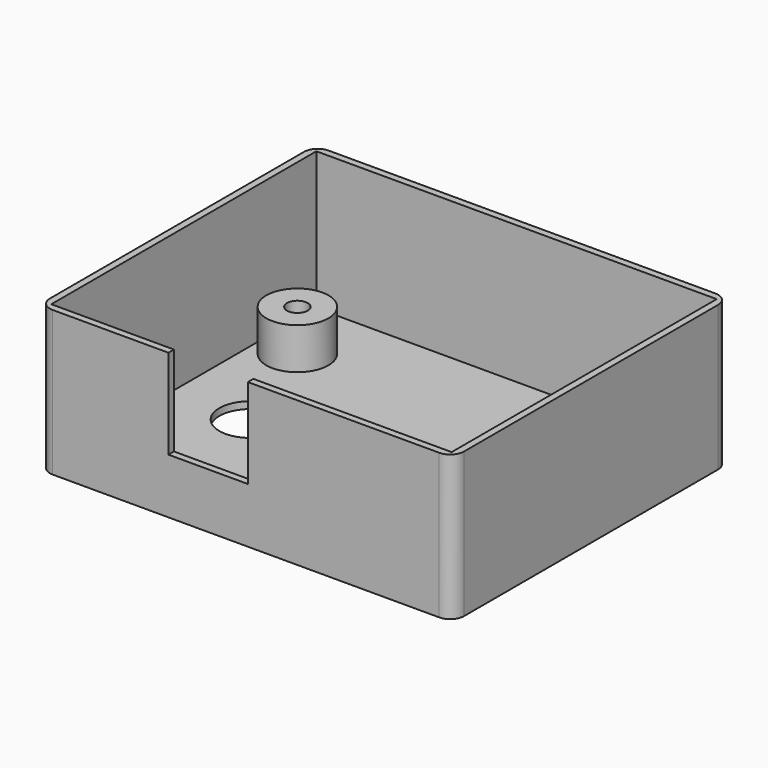
from build123d import *

# Parameters (mm, degrees)
F0_W      = 60
F0_H      = 50
F1_DEPTH  = 21
F2_W      = 58
F2_H      = 48
F3_DEPTH  = 20
F5_R      = 2
F6_R      = 4.5
F7_DEPTH  = 6
F10_W     = 11.5
F10_H     = 1
F11_DEPTH = 13
F12_W     = 2.5
F12_H     = 3.5
F13_DEPTH = 1
F14_R     = 4.5
F15_DEPTH = 1
F8_R      = 1.5
F16_DEPTH = 7
F9_R      = 1.5
F17_DEPTH = 7
F18_R     = 3.5
F18_R_2   = 1.5
F19_DEPTH = 1


with BuildPart() as f1:
    # F0 (on Top) → F1 (new body)
    with BuildSketch(Plane.XY):
        with Locations((-30, 25)):
            Rectangle(F0_W, F0_H)
    extrude(amount=F1_DEPTH)

    # F2 (on face) → F3 (cut)
    with BuildSketch(Plane.XY.offset(21)):
        with Locations((-30, 25)):
            Rectangle(F2_W, F2_H)
    extrude(amount=-F3_DEPTH, mode=Mode.SUBTRACT)

    # F5
    f5_edges = [f1.edges().sort_by_distance(p)[0] for p in [
        (-60, 50, 10.5),
        (0, 50, 10.5),
        (0, 0, 10.5),
        (-60, 0, 10.5),
    ]]
    fillet(f5_edges, radius=F5_R)

    # F6 (on face) → F7 (join)
    with BuildSketch(Plane.XY.offset(1)):
        with Locations((-22.1625890434, 6.5921834528)):
            Circle(F6_R)
        with Locations((-53.6625890434, 38.8921834528)):
            Circle(F6_R)
    extrude(amount=F7_DEPTH)

    # F10 (on face) → F11 (cut)
    with BuildSketch(Plane.XY.offset(21)):
        with Locations((-35.4789009094, 0.5)):
            Rectangle(F10_W, F10_H)
    extrude(amount=-F11_DEPTH, mode=Mode.SUBTRACT)

    # F12 (on face) → F13 (cut)
    with BuildSketch(Plane.XY.offset(1)):
        with Locations((-26.94821703, 11.3616460413)):
            Rectangle(F12_W, F12_H)
    extrude(amount=-F13_DEPTH, mode=Mode.SUBTRACT)

    # F14 (on face) → F15 (cut)
    with BuildSketch(Plane.XY.offset(1)):
        with Locations((-47.7578996122, 23)):
            Circle(F14_R)
    extrude(amount=-F15_DEPTH, mode=Mode.SUBTRACT)

    # F8 (on face) → F16 (cut)
    with BuildSketch(Plane.XY.offset(7)):
        with Locations((-53.6625890434, 38.8921834528)):
            Circle(F8_R)
    extrude(amount=-F16_DEPTH, mode=Mode.SUBTRACT)

    # F9 (on face) → F17 (cut)
    with BuildSketch(Plane.XY.offset(7)):
        with Locations((-22.1625890434, 6.5921834528)):
            Circle(F9_R)
    extrude(amount=-F17_DEPTH, mode=Mode.SUBTRACT)

    # F18 (on face) → F19 (cut)
    with BuildSketch(Plane(origin=(0, 0, 0), x_dir=(1, 0, 0), z_dir=(0, 0, -1))):
        with Locations((-22.1625890434, -6.5921834528)):
            Circle(F18_R)
        with Locations((-22.1625890434, -6.5921834528)):
            Circle(F18_R_2, mode=Mode.SUBTRACT)
        with Locations((-53.6625890434, -38.8921834528)):
            Circle(F18_R)
        with Locations((-53.6625890434, -38.8921834528)):
            Circle(F18_R_2, mode=Mode.SUBTRACT)
    extrude(amount=-F19_DEPTH, mode=Mode.SUBTRACT)


solid = f1.part
